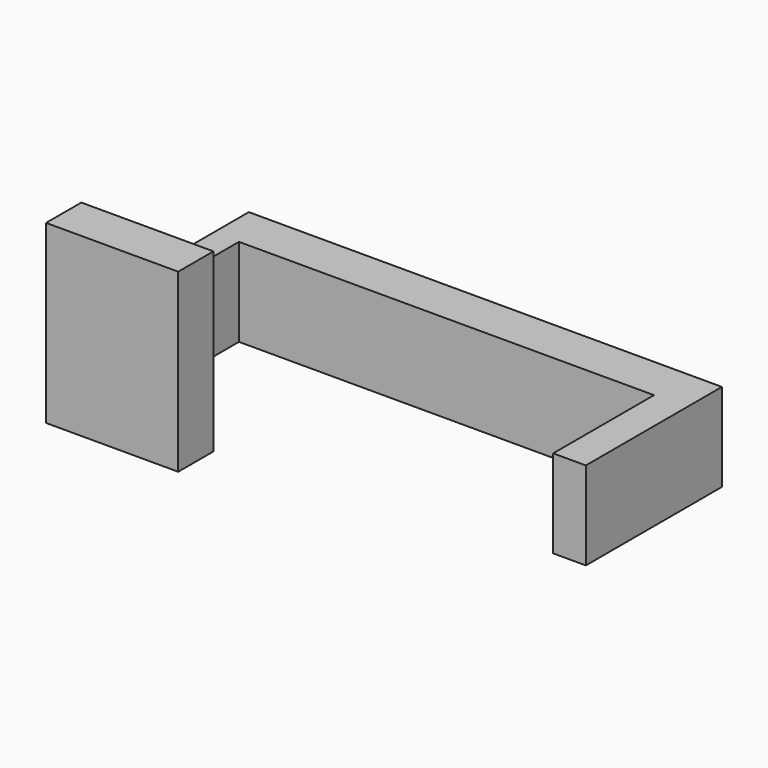
from build123d import *

# Parameters (mm, degrees)
F1_DEPTH      = 5
F3_DEPTH      = 5
F3_DEPTH_BACK = 5


# Not quite as in the source:
# - a feature names something its author has since deleted; it is built from what else it names


with BuildPart() as f1:
    # F0 (on Front) → F1 (new body)
    with BuildSketch(Plane.XZ):
        Polygon((0, 9.7736853705), (0, 0), (0, -10.2263146295), (15, -10.2263146295), (15, 9.7736853705), align=None)
    extrude(amount=F1_DEPTH)

    # F2 (on Top) → F3 (join, two sides)
    with BuildSketch(Plane.XY) as f3_sk:
        Polygon((7.0152175973, 15), (7.0152175973, 0), (9.8953448171, 0), (9.8953448171, 10), (57.0152175973, 10), (57.0152175973, -4.3088319683), (60.7257795132, -4.3088319683), (60.7257795132, 15), align=None)
    extrude(amount=F3_DEPTH)
    extrude(f3_sk.sketch, amount=-F3_DEPTH_BACK)


solid = f1.part
